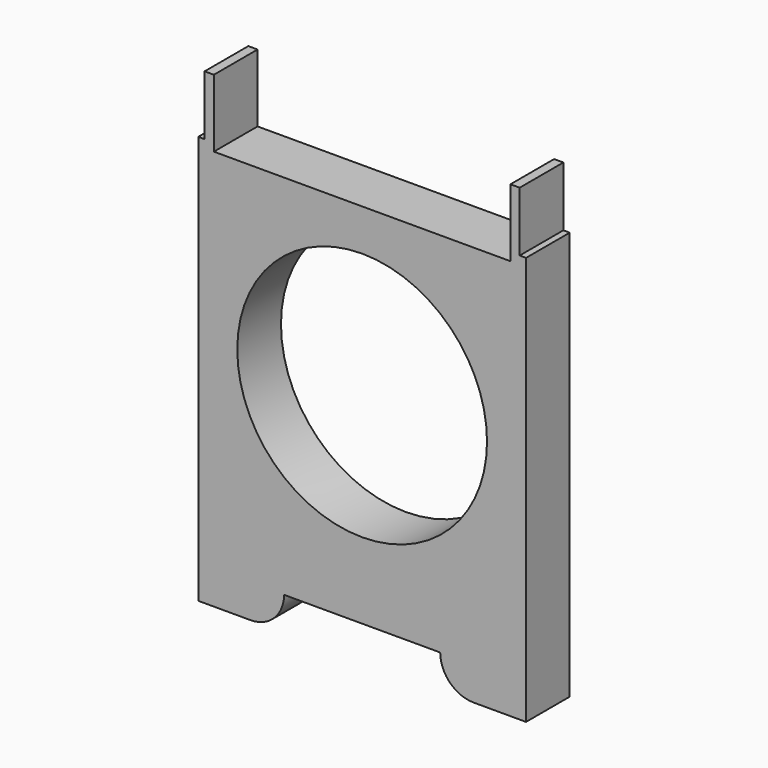
from build123d import *

# Parameters (mm, degrees)
F0_R        = 8
F1_DEPTH    = 3.5
F2_T4_DEPTH = 14.2095720734
F2_T9_DEPTH = 14.2095720734


# Not quite as in the source:
# - a fillet or chamfer that OpenCascade refuses, or shapes differently, is made with other operations: its cross-section is extruded or revolved along the edge and cut away or added


with BuildPart() as f1:
    # F0 (on Front) → F1 (new body)
    with BuildSketch(Plane.XZ):
        Polygon((5, -15), (10.5, -15), (10.5, 11.1734773964), (10.0929150358, 11.1734773964), (10.0929150358, 15), (9.5, 15), (9.5, 10.6615237892), (-9.5, 10.6615237892), (-9.5, 15), (-10.0929150358, 15), (-10.0929150358, 11.1734773964), (-10.5, 11.1734773964), (-10.5, -15), (-5, -15), (-5, -12.8721727654), (5, -12.8721727654), align=None)
        Circle(F0_R, mode=Mode.SUBTRACT)
    extrude(amount=F1_DEPTH)

    # F2: fillet of radius 2.1419144147 on 2 edges, made by hand


with BuildPart() as f2_tool2:
    # F2_s3 → F2_t4 (new body)
    with BuildSketch(Plane.XZ.offset(-5.3547860367)):
        with BuildLine():
            ThreePointArc((-7.1419144147, -15), (-5.6273522073, -14.3726477927), (-5, -12.8580855853))
            Line((-5, -12.8580855853), (-5, -15))
            Line((-5, -15), (-7.1419144147, -15))
        make_face()
    extrude(amount=F2_T4_DEPTH)

    split(bisect_by=Plane.XY.offset(-12.8721727654), keep=Keep.BOTTOM)


with BuildPart() as f1_1:
    add(f1.part)

    # F2_t1: cut F2_tool2
    add(f2_tool2.part, mode=Mode.SUBTRACT)


with BuildPart() as f2_tool7:
    # F2_s8 → F2_t9 (new body)
    with BuildSketch(Plane.XZ.offset(-5.3547860367)):
        with BuildLine():
            ThreePointArc((5, -12.8580855853), (5.6273522073, -14.3726477927), (7.1419144147, -15))
            Line((7.1419144147, -15), (5, -15))
            Line((5, -15), (5, -12.8580855853))
        make_face()
    extrude(amount=F2_T9_DEPTH)

    split(bisect_by=Plane.XY.offset(-12.8721727654), keep=Keep.BOTTOM)


with BuildPart() as f1_2:
    add(f1_1.part)

    # F2_t6: cut F2_tool7
    add(f2_tool7.part, mode=Mode.SUBTRACT)


solid = f1_2.part
